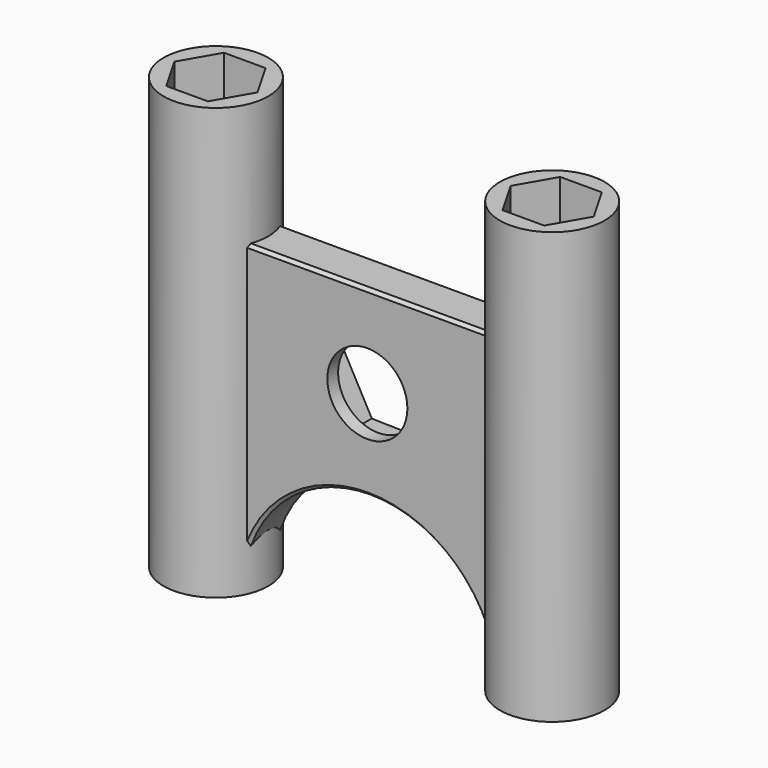
from build123d import *

# Parameters (mm, degrees)
F0_R          = 3.25
F1_DEPTH      = 3.5
F3_DEPTH      = 2.4
F4_R          = 4.25
F5_DEPTH      = 17.5
F5_DEPTH_BACK = 17.5
F6_SIZE       = 0.25


with BuildPart() as f1:
    # F0 (on Front) → F1 (new body)
    with BuildSketch(Plane.XZ):
        with BuildLine():
            Line((10.3391141687, -17.4996029254), (10.25, -7.5))
            Line((10.25, -7.5), (2.081973366, -7.5))
            ThreePointArc((2.081973366, -7.5), (7.9829074445, -11.0362777063), (10.3391141687, -17.4996029254))
        make_face()
        with BuildLine():
            Line((2.081973366, -7.5), (10.25, -7.5))
            Line((10.25, -7.5), (10.25, 7.5))
            Line((10.25, 7.5), (-10.25, 7.5))
            Line((-10.25, 7.5), (-10.25, -7.5))
            Line((-10.25, -7.5), (-1.9928591974, -7.5))
            ThreePointArc((-1.9928591974, -7.5), (0.0445570843, -7.2963797866), (2.081973366, -7.5))
        make_face()
        Circle(F0_R, mode=Mode.SUBTRACT)
        with BuildLine():
            ThreePointArc((-10.25, -17.4996029254), (-7.8937932759, -11.0362777063), (-1.9928591974, -7.5))
            Line((-1.9928591974, -7.5), (-10.25, -7.5))
            Line((-10.25, -7.5), (-10.25, -17.4996029254))
        make_face()
    extrude(amount=F1_DEPTH)

    # F2 (on Front) → F3 (cut)
    with BuildSketch(Plane.XZ):
        Polygon((-2.4370454627, -3.9929711461), (2.2394917178, -4.1070288539), (4.6765371804, -0.1140577078), (2.4370454627, 3.9929711461), (-2.2394917178, 4.1070288539), (-4.6765371804, 0.1140577078), align=None)
    extrude(amount=F3_DEPTH, mode=Mode.SUBTRACT)

    # F4 (on Top) → F5 (join, two sides)
    with BuildSketch(Plane.XY) as f5_sk:
        with Locations((13.65, -1.804011694)):
            Circle(F4_R)
        Polygon((17.0274990748, -1.804011694), (15.3387495374, -4.729011694), (11.9612504626, -4.729011694), (10.2725009252, -1.804011694), (11.9612504626, 1.120988306), (15.3387495374, 1.120988306), align=None, mode=Mode.SUBTRACT)
        with Locations((-13.65, -1.804011694)):
            Circle(F4_R)
        Polygon((-11.9612504626, -4.729011694), (-15.3387495374, -4.729011694), (-17.0274990748, -1.804011694), (-15.3387495374, 1.120988306), (-11.9612504626, 1.120988306), (-10.2725009252, -1.804011694), align=None, mode=Mode.SUBTRACT)
    extrude(amount=F5_DEPTH)
    extrude(f5_sk.sketch, amount=-F5_DEPTH_BACK)

    # F6
    f6_edges = [f1.edges().sort_by_distance(p)[0] for p in [
        (0, -3.5, 7.5),
        (0, 0, 7.5),
        (-0.094724, -3.5, -7.297322),
        (-0.101304, 0, -7.297413),
    ]]
    chamfer(f6_edges, length=F6_SIZE)


solid = f1.part
